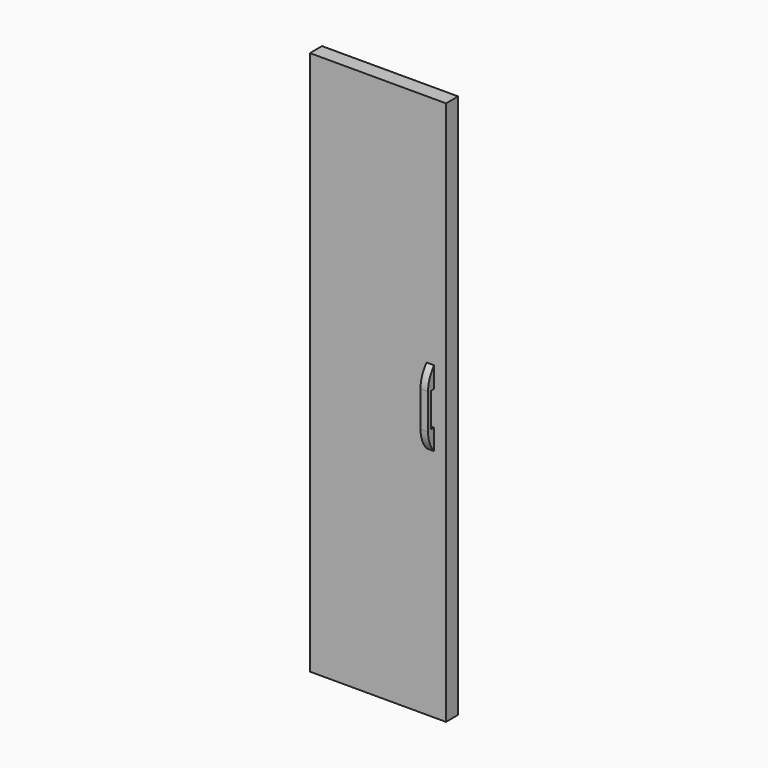
from build123d import *

# Parameters (mm, degrees)
F0_W        = 457.2
F0_H        = 1828.8
F1_DEPTH    = 50.8
F2_W        = 25.4
F2_H        = 254
F3_DEPTH    = 25.4
F4_T1_DEPTH = 361.4104165052
F5_W        = 12.7
F5_H        = 57.15
F6_DEPTH    = 417.2741922717


# Not quite as in the source:
# - a fillet or chamfer that OpenCascade refuses, or shapes differently, is made with other operations: its cross-section is extruded or revolved along the edge and cut away or added


with BuildPart() as f1:
    # F0 (on Front) → F1 (new body)
    with BuildSketch(Plane.XZ):
        Rectangle(F0_W, F0_H)
    extrude(amount=F1_DEPTH)

    # F2 (on face) → F3 (join)
    with BuildSketch(Plane.XZ.offset(50.8)):
        with Locations((175.9731922717, 0)):
            Rectangle(F2_W, F2_H)
    extrude(amount=F3_DEPTH)

    # F4: fillet of radius 101.6 on 2 edges, made by hand

    # F4_s2 → F4_t1 (cut)
    with BuildSketch(Plane.YZ.offset(-4.7320159809)):
        with BuildLine():
            ThreePointArc((-50.8, 127), (-69.6380976241, 95.7189411832), (-76.2, 59.797916699))
            Line((-76.2, 59.797916699), (-76.2, 127))
            Line((-76.2, 127), (-50.8, 127))
        make_face()
        with BuildLine():
            ThreePointArc((-50.8, -127), (-69.6380976241, -95.7189411832), (-76.2, -59.797916699))
            Line((-76.2, -59.797916699), (-76.2, -127))
            Line((-76.2, -127), (-50.8, -127))
        make_face()
    extrude(amount=F4_T1_DEPTH, mode=Mode.SUBTRACT)

    # F5 (on face) → F6 (cut, through all)
    with BuildSketch(Plane.YZ.offset(188.6731922717)):
        with Locations((-57.15, -28.575)):
            Rectangle(F5_W, F5_H)
        with Locations((-57.15, 28.575)):
            Rectangle(F5_W, F5_H)
    extrude(amount=-F6_DEPTH, mode=Mode.SUBTRACT)


solid = f1.part
